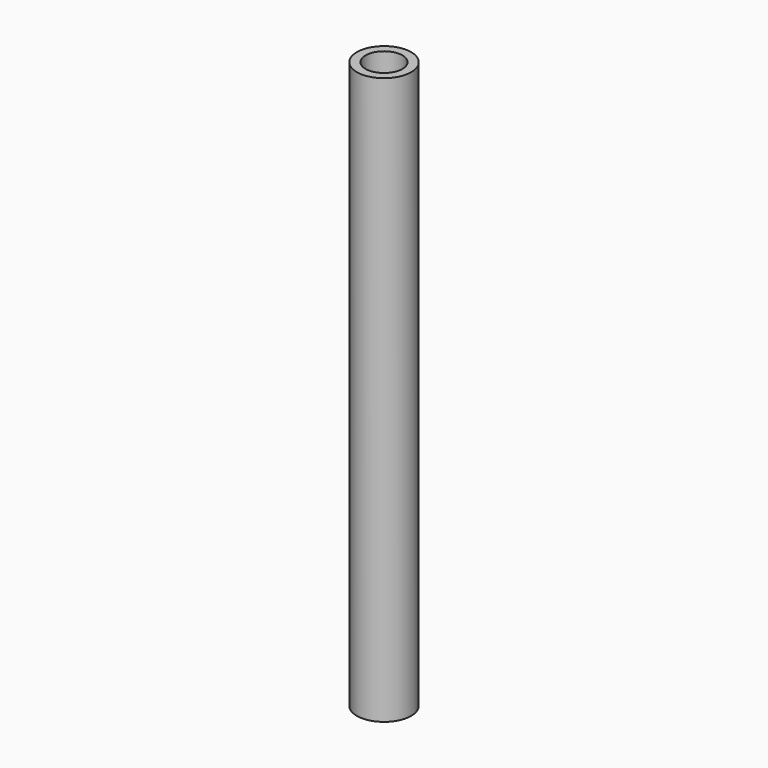
from build123d import *

# Parameters (mm, degrees)
F0_R     = 5.75
F0_R_2   = 3.9
F1_DEPTH = 120


# Not quite as in the source:
# - a feature names something its author has since deleted; it is built from what else it names


with BuildPart() as f1:
    # F0 (on Top) → F1 (new body)
    with BuildSketch(Plane.XY):
        Circle(F0_R)
        Circle(F0_R_2, mode=Mode.SUBTRACT)
    extrude(amount=F1_DEPTH)


solid = f1.part
